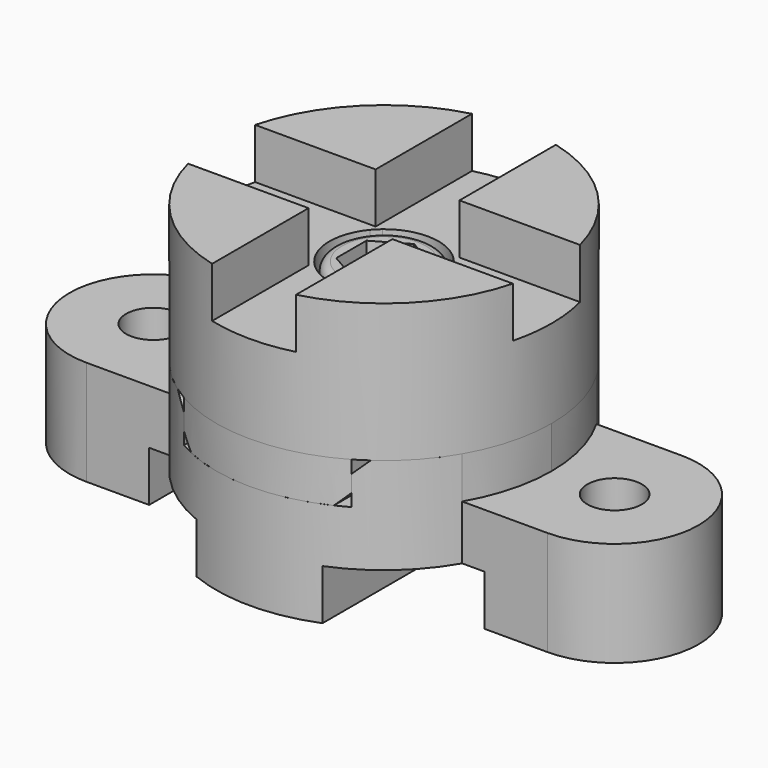
from build123d import *

# Parameters (mm, degrees)
F0_R      = 6.5
F1_DEPTH  = 35
F2_DEPTH  = 25
F3_W      = 40
F3_H      = 10
F3_W_2    = 25
F3_H_2    = 12
F4_DEPTH  = 50
F5_SIZE   = 3
F6_R      = 6.5
F7_DEPTH  = 10
F8_SIZE   = 3
F9_R      = 40
F10_DEPTH = 33
F12_DEPTH = 30
F13_DEPTH = 12
F14_DEPTH = 33.001
F17_SIZE  = 3
F19_DEPTH = 13


with BuildPart() as f1:
    # F0 (on Top) → F1 (new body)
    with BuildSketch(Plane.XY):
        with BuildLine():
            ThreePointArc((-34.6410161514, -20), (0, -40), (34.6410161514, -20))
            Line((34.6410161514, -20), (-34.6410161514, -20))
        make_face()
        with BuildLine():
            ThreePointArc((34.6410161514, -20), (38.6370330516, -10.3527618041), (40, 0))
            ThreePointArc((40, 0), (38.6370330516, 10.3527618041), (34.6410161514, 20))
            Line((34.6410161514, 20), (-34.6410161514, 20))
            ThreePointArc((-34.6410161514, 20), (-40, 0), (-34.6410161514, -20))
            Line((-34.6410161514, -20), (34.6410161514, -20))
        make_face()
        Circle(F0_R, mode=Mode.SUBTRACT)
        with BuildLine():
            Line((-34.6410161514, 20), (34.6410161514, 20))
            ThreePointArc((34.6410161514, 20), (0, 40), (-34.6410161514, 20))
        make_face()
    extrude(amount=F1_DEPTH)

    # F0 (on Top) → F2 (join)
    with BuildSketch(Plane.XY):
        with BuildLine():
            ThreePointArc((-34.6410161514, -20), (-40, 0), (-34.6410161514, 20))
            Line((-34.6410161514, 20), (-55, 20))
            ThreePointArc((-55, 20), (-75, 0), (-55, -20))
            Line((-55, -20), (-34.6410161514, -20))
        make_face()
        with Locations((-55, 0)):
            Circle(F0_R, mode=Mode.SUBTRACT)
        with BuildLine():
            ThreePointArc((34.6410161514, 20), (38.6370330516, 10.3527618041), (40, 0))
            ThreePointArc((40, 0), (38.6370330516, -10.3527618041), (34.6410161514, -20))
            Line((34.6410161514, -20), (55, -20))
            ThreePointArc((55, -20), (75, 0), (55, 20))
            Line((55, 20), (34.6410161514, 20))
        make_face()
        with Locations((55, 0)):
            Circle(F0_R, mode=Mode.SUBTRACT)
    extrude(amount=F2_DEPTH)

    # F3 (on Front) → F4 (cut, symmetric)
    with BuildSketch(Plane.XZ):
        with Locations((0, 30)):
            Rectangle(F3_W, F3_H)
        with Locations((-27.5, 6)):
            Rectangle(F3_W_2, F3_H_2)
        with Locations((27.5, 6)):
            Rectangle(F3_W_2, F3_H_2)
    extrude(amount=F4_DEPTH, both=True, mode=Mode.SUBTRACT)

    # F5
    f5_edges = [f1.edges().sort_by_distance(p)[0] for p in [
        (-20, 0, 35),
        (20, 0, 35),
    ]]
    chamfer(f5_edges, length=F5_SIZE)


with BuildPart() as f7:
    # F6 (on face) → F7 (new body, through all)
    with BuildSketch(Plane.XY.offset(25)):
        with BuildLine():
            Line((20, -34.6410161514), (20, 34.6410161514))
            ThreePointArc((20, 34.6410161514), (0, 40), (-20, 34.6410161514))
            Line((-20, 34.6410161514), (-20, -34.6410161514))
            ThreePointArc((-20, -34.6410161514), (0, -40), (20, -34.6410161514))
        make_face()
        Circle(F6_R, mode=Mode.SUBTRACT)
    extrude(amount=F7_DEPTH)

    # F8
    f8_edges = [f7.edges().sort_by_distance(p)[0] for p in [
        (20, 0, 25),
        (-20, 0, 25),
    ]]
    chamfer(f8_edges, length=F8_SIZE)

    # F9 (on face) → F10 (join)
    with BuildSketch(Plane.XY.offset(35)):
        Circle(F9_R)
    extrude(amount=F10_DEPTH)

    # F11 (on face) → F12 (cut)
    with BuildSketch(Plane.XY.offset(68)):
        with BuildLine():
            Line((-8.3066238629, 10), (8.3066238629, 10))
            ThreePointArc((8.3066238629, 10), (0, 13), (-8.3066238629, 10))
        make_face()
        with BuildLine():
            Line((10, -8.3066238629), (10, 8.3066238629))
            ThreePointArc((10, 8.3066238629), (9.1923881554, 9.1923881554), (8.3066238629, 10))
            Line((8.3066238629, 10), (-8.3066238629, 10))
            ThreePointArc((-8.3066238629, 10), (-9.1923881554, 9.1923881554), (-10, 8.3066238629))
            Line((-10, 8.3066238629), (-10, -8.3066238629))
            ThreePointArc((-10, -8.3066238629), (-9.1923881554, -9.1923881554), (-8.3066238629, -10))
            Line((-8.3066238629, -10), (8.3066238629, -10))
            ThreePointArc((8.3066238629, -10), (9.1923881554, -9.1923881554), (10, -8.3066238629))
        make_face()
        with BuildLine():
            Line((-10, -8.3066238629), (-10, 8.3066238629))
            ThreePointArc((-10, 8.3066238629), (-13, 0), (-10, -8.3066238629))
        make_face()
        with BuildLine():
            ThreePointArc((-8.3066238629, -10), (0, -13), (8.3066238629, -10))
            Line((8.3066238629, -10), (-8.3066238629, -10))
        make_face()
        with BuildLine():
            ThreePointArc((10, -8.3066238629), (12.2270192606, -4.4158804332), (13, 0))
            ThreePointArc((13, 0), (12.2270192606, 4.4158804332), (10, 8.3066238629))
            Line((10, 8.3066238629), (10, -8.3066238629))
        make_face()
    extrude(amount=-F12_DEPTH, mode=Mode.SUBTRACT)

    # F11 (on face) → F13 (cut)
    with BuildSketch(Plane.XY.offset(68)):
        with BuildLine():
            ThreePointArc((-8.3066238629, 10), (0, 13), (8.3066238629, 10))
            Line((8.3066238629, 10), (10, 10))
            Line((10, 10), (10, 38.7298334621))
            ThreePointArc((10, 38.7298334621), (5.0401716969, 39.681187851), (-4.8e-09, 40))
            ThreePointArc((-4.8e-09, 40), (-5.0401717017, 39.6811878504), (-10, 38.7298334621))
            Line((-10, 38.7298334621), (-10, 10))
            Line((-10, 10), (-8.3066238629, 10))
        make_face()
        with BuildLine():
            ThreePointArc((-10, -8.3066238629), (-13, 0), (-10, 8.3066238629))
            Line((-10, 8.3066238629), (-10, 10))
            Line((-10, 10), (-38.7298334621, 10))
            ThreePointArc((-38.7298334621, 10), (-39.6811878507, 5.0401716993), (-40, 0))
            ThreePointArc((-40, 0), (-39.6811878507, -5.0401716993), (-38.7298334621, -10))
            Line((-38.7298334621, -10), (-10, -10))
            Line((-10, -10), (-10, -8.3066238629))
        make_face()
        with BuildLine():
            ThreePointArc((-10, 8.3066238629), (-9.1923881554, 9.1923881554), (-8.3066238629, 10))
            Line((-8.3066238629, 10), (-10, 10))
            Line((-10, 10), (-10, 8.3066238629))
        make_face()
        with BuildLine():
            ThreePointArc((8.3066238629, 10), (9.1923881554, 9.1923881554), (10, 8.3066238629))
            Line((10, 8.3066238629), (10, 10))
            Line((10, 10), (8.3066238629, 10))
        make_face()
        with BuildLine():
            ThreePointArc((10, 8.3066238629), (12.2270192606, 4.4158804332), (13, 0))
            ThreePointArc((13, 0), (12.2270192606, -4.4158804332), (10, -8.3066238629))
            Line((10, -8.3066238629), (10, -10))
            Line((10, -10), (38.7298334621, -10))
            ThreePointArc((38.7298334621, -10), (39.6811878507, -5.0401716993), (40, 0))
            ThreePointArc((40, 0), (39.6811878507, 5.0401716993), (38.7298334621, 10))
            Line((38.7298334621, 10), (10, 10))
            Line((10, 10), (10, 8.3066238629))
        make_face()
        with BuildLine():
            Line((10, -10), (10, -8.3066238629))
            ThreePointArc((10, -8.3066238629), (9.1923881554, -9.1923881554), (8.3066238629, -10))
            Line((8.3066238629, -10), (10, -10))
        make_face()
        with BuildLine():
            Line((10, -10), (8.3066238629, -10))
            ThreePointArc((8.3066238629, -10), (0, -13), (-8.3066238629, -10))
            Line((-8.3066238629, -10), (-10, -10))
            Line((-10, -10), (-10, -38.7298334621))
            ThreePointArc((-10, -38.7298334621), (-5.0401716993, -39.6811878507), (0, -40))
            ThreePointArc((0, -40), (5.0401716993, -39.6811878507), (10, -38.7298334621))
            Line((10, -38.7298334621), (10, -10))
        make_face()
        with BuildLine():
            Line((-10, -10), (-8.3066238629, -10))
            ThreePointArc((-8.3066238629, -10), (-9.1923881554, -9.1923881554), (-10, -8.3066238629))
            Line((-10, -8.3066238629), (-10, -10))
        make_face()
    extrude(amount=-F13_DEPTH, mode=Mode.SUBTRACT)

    # F14 (cut, through all): a face of the model
    f14_faces = [f7.faces().sort_by_distance(p)[0] for p in [
        (0, 0, 35),
    ]]
    extrude(f14_faces, amount=-F14_DEPTH, mode=Mode.SUBTRACT)


with BuildPart() as f16:
    # F15 (on Front) → F16 (revolve)
    with BuildSketch(Plane.XZ):
        with BuildLine():
            Line((10, 56), (0, 56))
            Line((0, 56), (0, 8))
            Line((0, 8), (6.5, 8))
            Line((6.5, 8), (6.5, 38))
            Line((6.5, 38), (10, 38))
            ThreePointArc((10, 38), (11.4142135624, 38.5857864376), (12, 40))
            Line((12, 40), (12, 54))
            ThreePointArc((12, 54), (11.4142135624, 55.4142135624), (10, 56))
        make_face()
    revolve(axis=Axis((0, 0, 32), (0, 0, 1)))

    # F17
    f17_edges = [f16.edges().sort_by_distance(p)[0] for p in [
        (-6.5, 0, 8),
    ]]
    chamfer(f17_edges, length=F17_SIZE)

    # F18 (on face) → F19 (cut)
    with BuildSketch(Plane.XY.offset(56)):
        Polygon((7.7942286341, -4.5), (7.7942286341, 4.5), (0, 9), (-7.7942286341, 4.5), (-7.7942286341, -4.5), (0, -9), align=None)
    extrude(amount=-F19_DEPTH, mode=Mode.SUBTRACT)


solid = Compound([f1.part, f7.part, f16.part])
